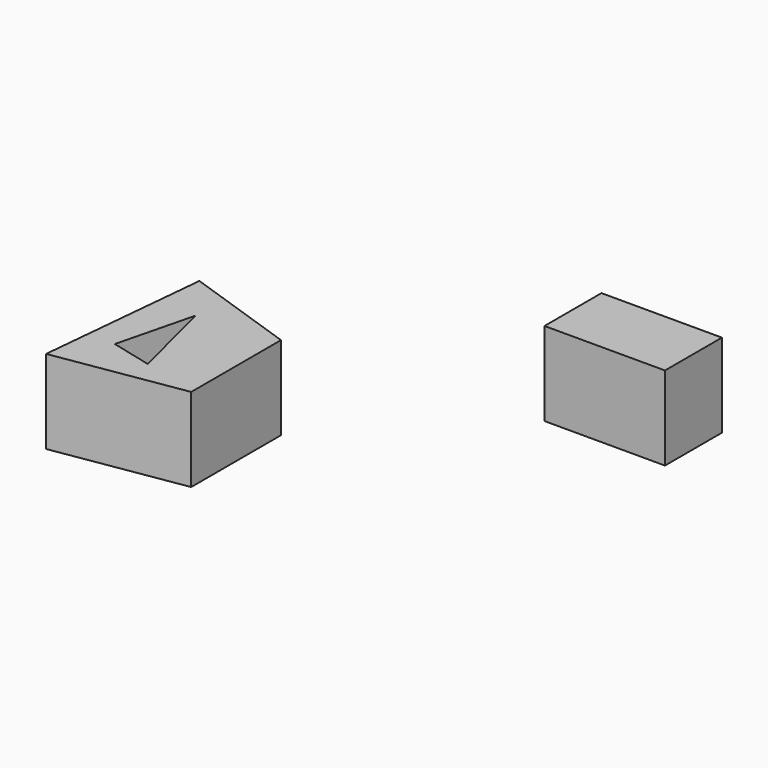
from build123d import *

# Parameters (mm, degrees)
F1_DEPTH = 25.4
F0_W     = 36.5379918367
F0_H     = 21.5906333178
F2_DEPTH = 25.4


# Not quite as in the source:
# - the program builds the solid bodies; features that only make, move or delete a surface that nothing else refers to are left out


with BuildPart() as f1:
    # F0 (on Top) → F1 (new body)
    with BuildSketch(Plane.XY):
        Polygon((-20.9524314851, -29.0797241032), (-54.9991987646, -17.4539964646), (-59.9816553295, -69.3545565009), (-20.9524314851, -63.1264895201), align=None)
        Polygon((-50.4319518805, -55.2375987172), (-44.6190871298, -31.9861508906), (-37.9269696142, -58.3638457864), align=None, mode=Mode.SUBTRACT)
    extrude(amount=F1_DEPTH)


with BuildPart() as f2:
    # F0 (on Top) → F2 (new body)
    with BuildSketch(Plane.XY):
        with Locations((41.5204456076, 26.3654785231)):
            Rectangle(F0_W, F0_H)
    extrude(amount=F2_DEPTH)


solid = Compound([f1.part, f2.part])
